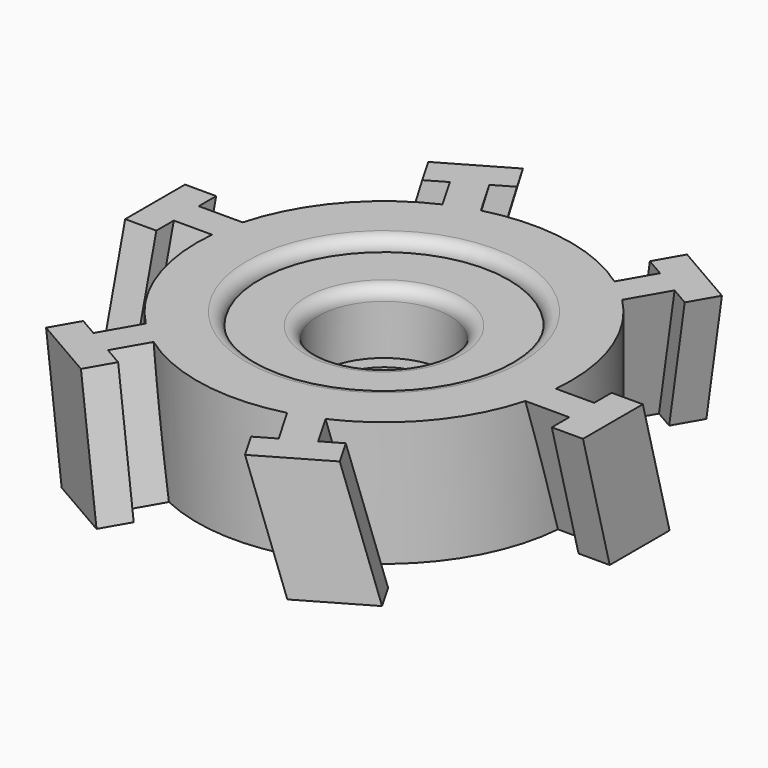
from build123d import *

# Parameters (mm, degrees)
F0_R      = 15
F0_R_2    = 10
F2_DEPTH  = 10
F1_W      = 6
F1_H      = 2.5
F7_COUNT  = 6
F0_R_3    = 5.25
F0_R_4    = 4
F9_DEPTH  = 4
F10_DEPTH = 9
F11_R     = 0.99999


# Not quite as in the source:
# - a fillet or chamfer is up to 0.001 mm smaller than in the source, because OpenCascade refuses the exact size


with BuildPart() as f2:
    # F0 (on Top) → F2 (new body)
    with BuildSketch(Plane.XY):
        Circle(F0_R)
        Circle(F0_R_2, mode=Mode.SUBTRACT)
    extrude(amount=F2_DEPTH)

    # F6: sweep along a path in F5
    with BuildLine(Plane.YZ.offset(-12)) as f6_path:
        Line((-1.25, 0), (1.4294919243, 10))
    # F1 (on Top) → F6 (sweep)
    with BuildSketch(Plane.XY):
        Polygon((-18, -1.25), (-18, 1.25), (-18, 3), (-20.5, 3), (-20.5, -3), (-18, -3), align=None)
        with Locations((-15, 0)):
            Rectangle(F1_W, F1_H)
    sweep(path=f6_path.line)

    # F7: F2 ×6 about axis
    f7_axis = Axis((0, 0, 0), (0, 0, 1))


with BuildPart() as f2_1:
    add(f2.part)
    for i in range(1, F7_COUNT):
        add(f2.part.rotate(f7_axis, i * 360 / F7_COUNT))



with BuildPart() as f9:
    # F0 (on Top) → F9 (new body)
    with BuildSketch(Plane.XY):
        Circle(F0_R_3)
        Circle(F0_R_4, mode=Mode.SUBTRACT)
    extrude(amount=F9_DEPTH)


with BuildPart() as f2_2:
    add(f2_1.part)

    add(f9.part)  # F10 merges F9
    # F0 (on Top) → F10 (join)
    with BuildSketch(Plane.XY):
        Circle(F0_R_2)
        Circle(F0_R_3, mode=Mode.SUBTRACT)
    extrude(amount=F10_DEPTH)

    # F11 (radius 1 in the source; OpenCascade refuses exactly that, so slightly less here)
    f11_edges = [f2_2.edges().sort_by_distance(p)[0] for p in [
        (-10, 0, 10),
        (-5.25, 0, 9),
    ]]
    fillet(f11_edges, radius=F11_R)


solid = f2_2.part
